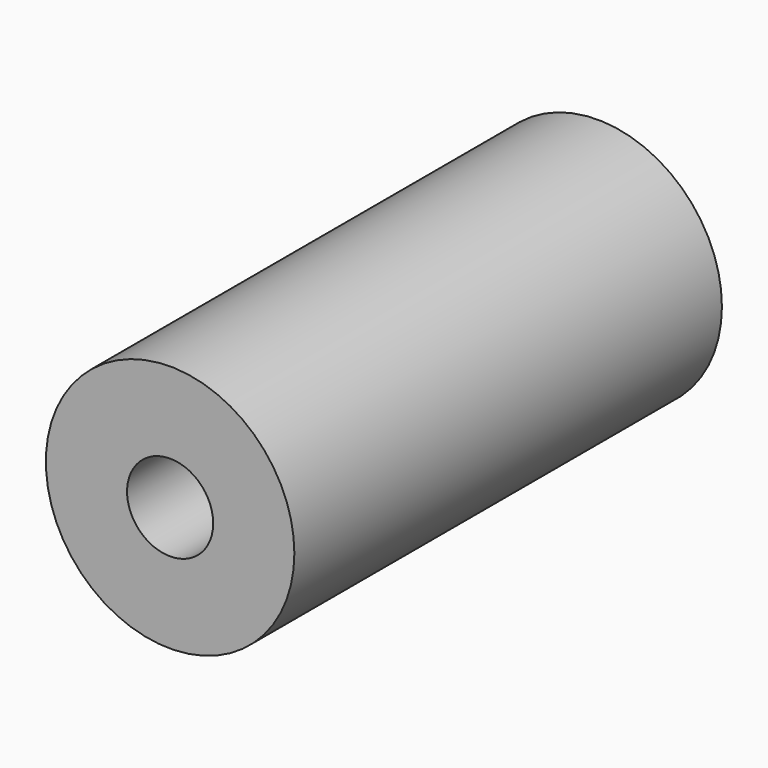
from build123d import *

# Parameters (mm, degrees)
F0_R          = 23.6201773587
F0_R_2        = 8.1878472109
F1_DEPTH      = 50.8
F1_DEPTH_BACK = 50.8


# Not quite as in the source:
# - the program builds the solid bodies; features that only make, move or delete a surface that nothing else refers to are left out


with BuildPart() as f1:
    # F0 (on Front) → F1 (new body, two sides)
    with BuildSketch(Plane.XZ) as f1_sk:
        Circle(F0_R)
        Circle(F0_R_2, mode=Mode.SUBTRACT)
    extrude(amount=F1_DEPTH)
    extrude(f1_sk.sketch, amount=-F1_DEPTH_BACK)


solid = f1.part
